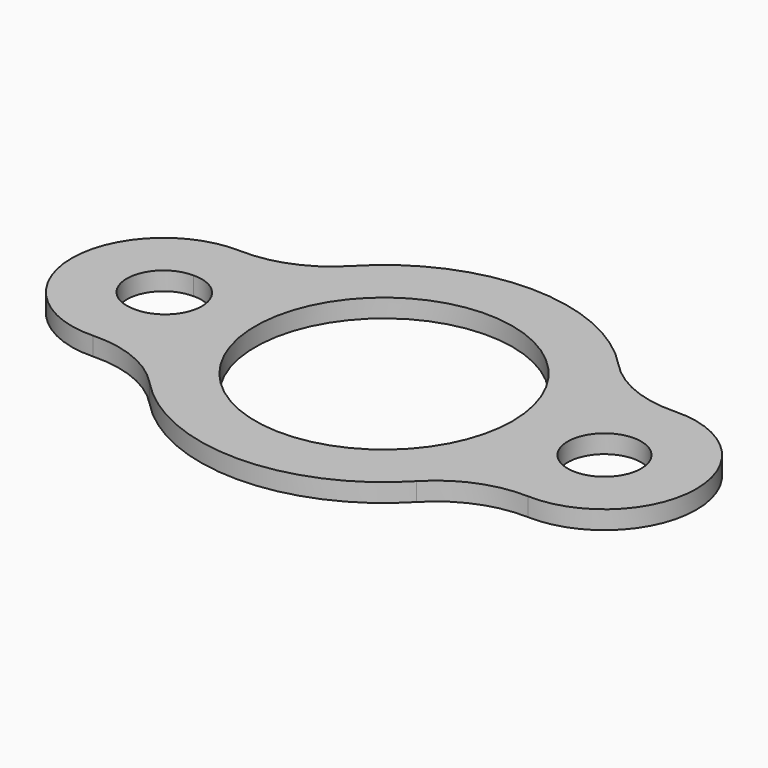
from build123d import *

# Parameters (mm, degrees)
F0_R     = 44.45
F0_R_2   = 12.7
F2_DEPTH = 6.35


# Not quite as in the source:
# - a feature of the source that left no trace in its solid (it failed there, or was rolled back) is left out


with BuildPart() as f2:
    # F0 (on Top) → F2 (new body)
    with BuildSketch(Plane.XY):
        with BuildLine():
            ThreePointArc((46.13671875, -43.6308741946), (59.3475236203, -34.5646316236), (75.1176136364, -31.7315448688))
            ThreePointArc((75.1176136364, -31.7315448688), (107.95, 0), (75.1176136364, 31.7315448688))
            ThreePointArc((75.1176136364, 31.7315448688), (59.3475236203, 34.5646316236), (46.13671875, 43.6308741946))
            ThreePointArc((46.13671875, 43.6308741946), (0, 63.5), (-46.13671875, 43.6308741946))
            ThreePointArc((-46.13671875, 43.6308741946), (-59.3475236203, 34.5646316236), (-75.1176136364, 31.7315448688))
            ThreePointArc((-75.1176136364, 31.7315448688), (-107.95, 0), (-75.1176136364, -31.7315448688))
            ThreePointArc((-75.1176136364, -31.7315448688), (-59.3475236203, -34.5646316236), (-46.13671875, -43.6308741946))
            ThreePointArc((-46.13671875, -43.6308741946), (0, -63.5), (46.13671875, -43.6308741946))
        make_face()
        with BuildLine():
            ThreePointArc((-75.9357507288, 12.6972505812), (-66.7851626656, 9.0732013574), (-62.9715014577, 0))
            ThreePointArc((-62.9715014577, 0), (-66.7851626656, -9.0732013574), (-75.9357507288, -12.6972505812))
            ThreePointArc((-75.9357507288, -12.6972505812), (-88.9, 0), (-75.9357507288, 12.6972505812))
        make_face(mode=Mode.SUBTRACT)
        Circle(F0_R, mode=Mode.SUBTRACT)
        with Locations((76.2, 0)):
            Circle(F0_R_2, mode=Mode.SUBTRACT)
    extrude(amount=F2_DEPTH)


solid = f2.part
